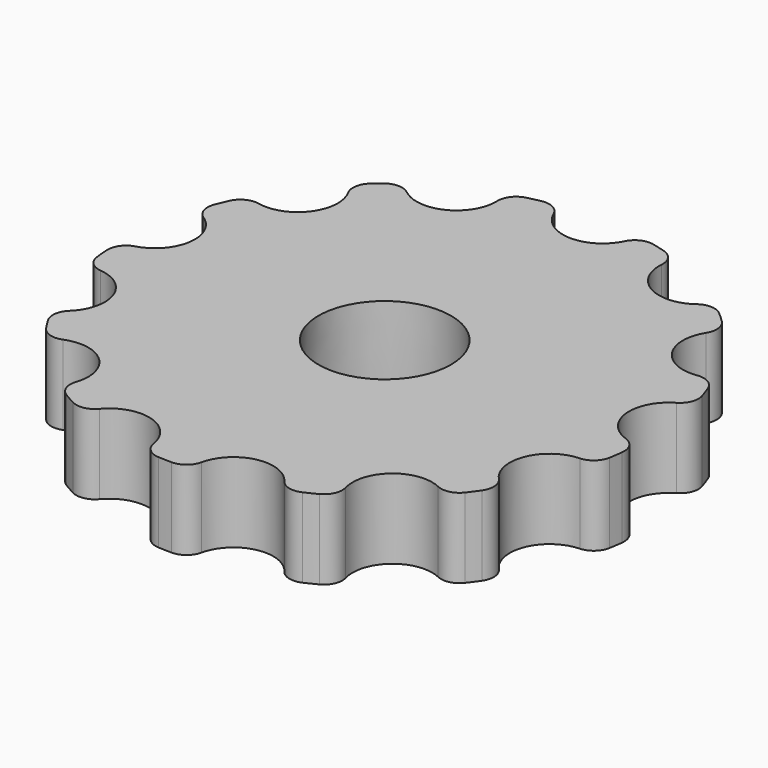
from build123d import *

# Parameters (mm, degrees)
F0_R     = 1.4
F1_DEPTH = 3
F3_R     = 3.5
F3_R_2   = 1.4
F4_DEPTH = 2
F5_R     = 2.5
F6_DEPTH = 3.2
F6_TAPER = -2
F7_R     = 0.7
F8_R     = 0.99999


# Not quite as in the source:
# - a fillet or chamfer is up to 0.001 mm smaller than in the source, because OpenCascade refuses the exact size


with BuildPart() as f1:
    # F0 (on Top) → F1 (new body)
    with BuildSketch(Plane.XY):
        with BuildLine():
            ThreePointArc((9.9850004133, -0.5475095853), (8.4613796466, 0.8093543575), (9.7001504704, 2.4304486935))
            ThreePointArc((9.7001504704, 2.4304486935), (9.4357647354, 3.3115470492), (9.0915303388, 4.1646219635))
            ThreePointArc((9.0915303388, 4.1646219635), (7.1113692422, 4.6560098261), (7.4528610453, 6.6674479556))
            ThreePointArc((7.4528610453, 6.6674479556), (6.80863075, 7.3241072705), (6.1067834976, 7.9187874901))
            ThreePointArc((6.1067834976, 7.9187874901), (4.1255680829, 7.4316679146), (3.4912293072, 9.3707693347))
            ThreePointArc((3.4912293072, 9.3707693347), (2.6153433482, 9.6519417306), (1.7173254612, 9.8514361014))
            ThreePointArc((1.7173254612, 9.8514361014), (0.1907842596, 8.4978586342), (-1.2734714925, 9.918582074))
            ThreePointArc((-1.2734714925, 9.918582074), (-2.1795376882, 9.7595909477), (-3.0671598922, 9.5180108319))
            ThreePointArc((-3.0671598922, 9.5180108319), (-3.7878846605, 7.6093317577), (-5.7452423622, 8.1848756985))
            ThreePointArc((-5.7452423622, 8.1848756985), (-6.4230450902, 7.6644955326), (-7.0539459688, 7.0881482963))
            ThreePointArc((-7.0539459688, 7.0881482963), (-6.8295942728, 5.0603005908), (-8.8349042364, 4.6844921959))
            ThreePointArc((-8.8349042364, 4.6844921959), (-9.2279972225, 3.8527999249), (-9.5429997466, 2.9885039461))
            ThreePointArc((-9.5429997466, 2.9885039461), (-8.4002559326, 1.2983452034), (-9.9999486142, 0.032057983))
            ThreePointArc((-9.9999486142, 0.032057983), (-9.9605830494, -0.8870091971), (-9.8369276314, -1.7985702027))
            ThreePointArc((-9.8369276314, -1.7985702027), (-8.038651031, -2.7622616825), (-8.8647575612, -4.6277503586))
            ThreePointArc((-8.8647575612, -4.6277503586), (-8.4019884988, -5.4227842725), (-7.8681189422, -6.1719287351))
            ThreePointArc((-7.8681189422, -6.1719287351), (-5.827957636, -6.1874800843), (-5.6904530873, -8.2230616963))
            ThreePointArc((-5.6904530873, -8.2230616963), (-4.9107288537, -8.7111848864), (-4.0894483565, -9.125591057))
            ThreePointArc((-4.0894483565, -9.125591057), (-2.276689888, -8.1894250808), (-1.2072037065, -9.926865528))
            ThreePointArc((-1.2072037065, -9.926865528), (-0.2898801541, -9.9957975918), (0.6298964632, -9.9801418049))
            ThreePointArc((0.6298964632, -9.9801418049), (1.7982728255, -8.3075998246), (3.553732375, -9.3472448458))
            ThreePointArc((3.553732375, -9.3472448458), (4.3976481483, -8.9811297042), (5.204349522, -8.5390131779))
            ThreePointArc((5.204349522, -8.5390131779), (5.4595883267, -6.5148212027), (7.4972221439, -6.6175267377))
            ThreePointArc((7.4972221439, -6.6175267377), (8.0736086443, -5.9005799256), (8.5816735129, -5.1337003923))
            ThreePointArc((8.5816735129, -5.1337003923), (7.8650635241, -3.2234726247), (9.7161654504, -2.3656138612))
            ThreePointArc((9.7161654504, -2.3656138612), (9.8924395316, -1.4627508718), (9.9850004133, -0.5475095853))
        make_face()
        Circle(F0_R, mode=Mode.SUBTRACT)
    extrude(amount=F1_DEPTH)

    # F3 (on face) → F4 (join)
    with BuildSketch(Plane(origin=(0, 0, 0), x_dir=(1, 0, 0), z_dir=(0, 0, -1))):
        Circle(F3_R)
        Circle(F3_R_2, mode=Mode.SUBTRACT)
    extrude(amount=F4_DEPTH)

    # F5 (on face) → F6 (cut)
    with BuildSketch(Plane.XY.offset(3)):
        Circle(F5_R)
    extrude(amount=-F6_DEPTH, taper=F6_TAPER, mode=Mode.SUBTRACT)

    # F7
    f7_edges = [f1.edges().sort_by_distance(p)[0] for p in [
        (-8.864758, -4.62775, 1.5),
        (-5.690453, -8.223062, 1.5),
        (-1.207204, -9.926866, 1.5),
        (3.553732, -9.347245, 1.5),
        (-9.999949, 0.032058, 1.5),
        (-8.834904, 4.684492, 1.5),
        (-5.745242, 8.184876, 1.5),
        (-1.273471, 9.918582, 1.5),
        (3.491229, 9.370769, 1.5),
        (7.452861, 6.667448, 1.5),
        (9.70015, 2.430449, 1.5),
        (9.716165, -2.365614, 1.5),
        (7.497222, -6.617527, 1.5),
        (5.20435, -8.539013, 1.5),
        (8.581674, -5.1337, 1.5),
        (0.629896, -9.980142, 1.5),
        (9.985, -0.54751, 1.5),
        (-4.089448, -9.125591, 1.5),
        (9.09153, 4.164622, 1.5),
        (-7.868119, -6.171929, 1.5),
        (6.106783, 7.918787, 1.5),
        (-9.836928, -1.79857, 1.5),
        (1.717325, 9.851436, 1.5),
        (-9.543, 2.988504, 1.5),
        (-3.06716, 9.518011, 1.5),
        (-7.053946, 7.088148, 1.5),
    ]]
    fillet(f7_edges, radius=F7_R)

    # F8 (radius 1 in the source; OpenCascade refuses exactly that, so slightly less here)
    f8_edges = [f1.edges().sort_by_distance(p)[0] for p in [
        (-3.5, 0, 0),
        (-3.5, 0, -2),
    ]]
    fillet(f8_edges, radius=F8_R)


solid = f1.part
